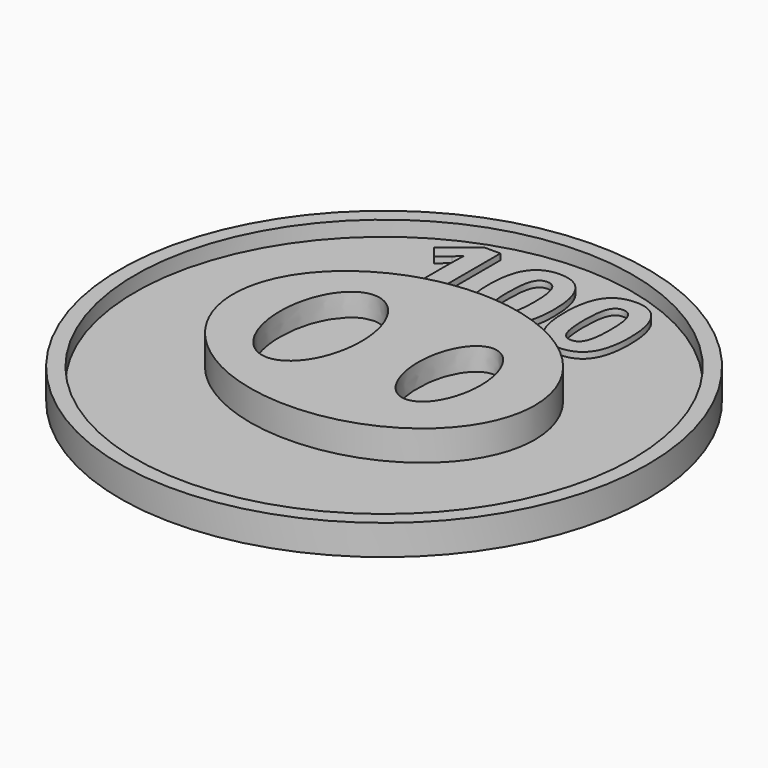
from build123d import *

# Parameters (mm, degrees)
F0_R         = 17.5
F0_R_2       = 16.5
F1_DEPTH     = 2
F2_DEPTH     = 3
F3_DEPTH     = 1.5
F4_DEPTH     = 1
F5_TEXT_SIZE = 8.8054631919
F6_DEPTH     = 0.4


# Not quite as in the source:
# - Text() gives the source's letters only with a copy of the font that has no kerning and outlines rounded to 1/6400 em; it was checked with that copy


with BuildPart() as f1:
    # F0 (on Top) → F1 (new body)
    with BuildSketch(Plane.XY):
        Circle(F0_R)
        Circle(F0_R_2, mode=Mode.SUBTRACT)
    extrude(amount=F1_DEPTH)

    # F0 (on Top) → F4 (join)
    with BuildSketch(Plane.XY):
        Circle(F0_R_2)
        with BuildLine():
            add(Edge.make_bspline(
                [(10, 0), (10, 13.8564064606), (-5, 6.9282032303), (-20, 0), (-5, -6.9282032303), (10, -13.8564064606), (10, 0)],
                knots=[0, 0, 0, 2.0943951024, 2.0943951024, 4.1887902048, 4.1887902048, 6.2831853072, 6.2831853072, 6.2831853072], degree=2, weights=[1, 0.5, 1, 0.5, 1, 0.5, 1]))
        make_face(mode=Mode.SUBTRACT)
    extrude(amount=F4_DEPTH)

    # F5 (on face) → F6 (join)
    with BuildSketch(Plane.XY.offset(1)):
        with Locations((-7.5987427848, 8.3061959594)):
            Text('100', F5_TEXT_SIZE, font='Open Sans', font_style=FontStyle.BOLD, text_align=(TextAlign.LEFT, TextAlign.BOTTOM))
    extrude(amount=F6_DEPTH)


with BuildPart() as f2:
    # F0 (on Top) → F2 (new body)
    with BuildSketch(Plane.XY):
        with BuildLine():
            add(Edge.make_bspline(
                [(10, 0), (10, 13.8564064606), (-5, 6.9282032303), (-20, 0), (-5, -6.9282032303), (10, -13.8564064606), (10, 0)],
                knots=[0, 0, 0, 2.0943951024, 2.0943951024, 4.1887902048, 4.1887902048, 6.2831853072, 6.2831853072, 6.2831853072], degree=2, weights=[1, 0.5, 1, 0.5, 1, 0.5, 1]))
        make_face()
        with BuildLine():
            add(Edge.make_bspline(
                [(-4.2034685612, -4.4573703781), (0.4776467724, -4.4573703781), (-1.8629108944, 2.228685189), (-4.2034685612, 8.9147407562), (-6.5440262279, 2.228685189), (-8.8845838947, -4.4573703781), (-4.2034685612, -4.4573703781)],
                knots=[0, 0, 0, 2.0943951024, 2.0943951024, 4.1887902048, 4.1887902048, 6.2831853072, 6.2831853072, 6.2831853072], degree=2, weights=[1, 0.5, 1, 0.5, 1, 0.5, 1]))
        make_face(mode=Mode.SUBTRACT)
        with BuildLine():
            add(Edge.make_bspline(
                [(4.3287393637, -3.6316728219), (7.9188687367, -3.6316728219), (6.1238040502, 1.815836411), (4.3287393637, 7.2633456439), (2.5336746772, 1.815836411), (0.7386099907, -3.6316728219), (4.3287393637, -3.6316728219)],
                knots=[0, 0, 0, 2.0943951024, 2.0943951024, 4.1887902048, 4.1887902048, 6.2831853072, 6.2831853072, 6.2831853072], degree=2, weights=[1, 0.5, 1, 0.5, 1, 0.5, 1]))
        make_face(mode=Mode.SUBTRACT)
    extrude(amount=F2_DEPTH)


with BuildPart() as f3:
    # F0 (on Top) → F3 (new body)
    with BuildSketch(Plane.XY):
        with BuildLine():
            add(Edge.make_bspline(
                [(-4.2034685612, -4.4573703781), (0.4776467724, -4.4573703781), (-1.8629108944, 2.228685189), (-4.2034685612, 8.9147407562), (-6.5440262279, 2.228685189), (-8.8845838947, -4.4573703781), (-4.2034685612, -4.4573703781)],
                knots=[0, 0, 0, 2.0943951024, 2.0943951024, 4.1887902048, 4.1887902048, 6.2831853072, 6.2831853072, 6.2831853072], degree=2, weights=[1, 0.5, 1, 0.5, 1, 0.5, 1]))
        make_face()
    extrude(amount=F3_DEPTH)


with BuildPart() as f3b:
    # F0 (on Top) → F3, piece 2 (new body)
    with BuildSketch(Plane.XY):
        with BuildLine():
            add(Edge.make_bspline(
                [(4.3287393637, -3.6316728219), (7.9188687367, -3.6316728219), (6.1238040502, 1.815836411), (4.3287393637, 7.2633456439), (2.5336746772, 1.815836411), (0.7386099907, -3.6316728219), (4.3287393637, -3.6316728219)],
                knots=[0, 0, 0, 2.0943951024, 2.0943951024, 4.1887902048, 4.1887902048, 6.2831853072, 6.2831853072, 6.2831853072], degree=2, weights=[1, 0.5, 1, 0.5, 1, 0.5, 1]))
        make_face()
    extrude(amount=F3_DEPTH)


solid = Compound([f1.part, f2.part, f3.part, f3b.part])
